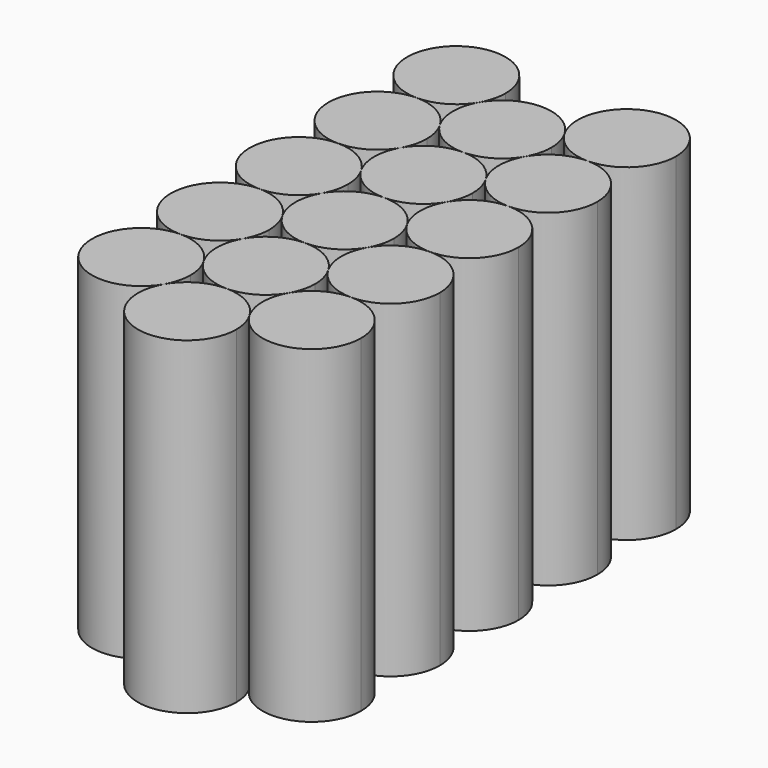
from build123d import *

# Parameters (mm, degrees)
F1_DEPTH = 70


# Not quite as in the source:
# - a feature names something its author has since deleted; it is built from what else it names


with BuildPart() as f1:
    # F0 (on Top) → F1 (new body)
    with BuildSketch(Plane.XY):
        with BuildLine():
            ThreePointArc((-9.0932666667, 5.2500001264), (-2.7176000441, -10.1422211571), (10.5, 0))
            ThreePointArc((10.5, 0), (10.1422211824, 2.71759995), (9.0932667642, 5.2499999577))
            ThreePointArc((9.0932667642, 5.2499999577), (5.2500000295, 9.0932667227), (1.93e-08, 10.5))
            ThreePointArc((1.93e-08, 10.5), (-5.2499999284, 9.0932667811), (-9.0932666667, 5.2500001264))
        make_face()
    extrude(amount=F1_DEPTH)


with BuildPart() as f1b:
    # F0 (on Top) → F1, piece 2 (new body)
    with BuildSketch(Plane.XY):
        with BuildLine():
            ThreePointArc((9.0932667504, 15.7500000185), (7.6865334795, 10.4999999862), (9.0932667642, 5.2499999577))
            ThreePointArc((9.0932667642, 5.2499999577), (20.9041334767, 0.3577788303), (28.6865334795, 10.5))
            ThreePointArc((28.6865334795, 10.5), (25.6111546956, 17.9246211888), (18.1865335182, 21))
            ThreePointArc((18.1865335182, 21), (12.9365335055, 19.5932667547), (9.0932667504, 15.7500000185))
        make_face()
    extrude(amount=F1_DEPTH)


with BuildPart() as f1c:
    # F0 (on Top) → F1, piece 3 (new body)
    with BuildSketch(Plane.XY):
        with BuildLine():
            ThreePointArc((-18.1865334408, 21), (-27.2798001924, 5.2499999535), (-9.0932666667, 5.2500001264))
            ThreePointArc((-9.0932666667, 5.2500001264), (-8.0443122845, 7.7824000969), (-7.6865334795, 10.5))
            ThreePointArc((-7.6865334795, 10.5), (-8.0443122981, 13.2175999536), (-9.0932667191, 15.7499999643))
            ThreePointArc((-9.0932667191, 15.7499999643), (-12.9365334449, 19.5932667197), (-18.1865334408, 21))
        make_face()
    extrude(amount=F1_DEPTH)


with BuildPart() as f1d:
    # F0 (on Top) → F1, piece 4 (new body)
    with BuildSketch(Plane.XY):
        with BuildLine():
            ThreePointArc((-9.0932667191, 15.7499999643), (-5.2499999738, 11.9067332451), (1.93e-08, 10.5))
            ThreePointArc((1.93e-08, 10.5), (5.2500000176, 11.9067332704), (9.0932667504, 15.7500000185))
            ThreePointArc((9.0932667504, 15.7500000185), (10.1422211788, 18.2824000367), (10.5, 21))
            ThreePointArc((10.5, 21), (10.1422211707, 23.7175999935), (9.0932667191, 26.2500000357))
            ThreePointArc((9.0932667191, 26.2500000357), (5.2499999989, 30.0932667404), (3.87e-08, 31.5))
            ThreePointArc((3.87e-08, 31.5), (-5.2500000363, 30.0932667188), (-9.093266801, 26.2499998939))
            ThreePointArc((-9.093266801, 26.2499998939), (-10.5, 20.9999999181), (-9.0932667191, 15.7499999643))
        make_face()
    extrude(amount=F1_DEPTH)


with BuildPart() as f1e:
    # F0 (on Top) → F1, piece 5 (new body)
    with BuildSketch(Plane.XY):
        with BuildLine():
            ThreePointArc((-18.1865333975, 42), (-28.6865334795, 31.5000000216), (-18.1865334408, 21))
            ThreePointArc((-18.1865334408, 21), (-12.9365335158, 22.4067332393), (-9.093266801, 26.2499998939))
            ThreePointArc((-9.093266801, 26.2499998939), (-8.0443123193, 28.7823999672), (-7.6865334795, 31.5))
            ThreePointArc((-7.6865334795, 31.5), (-8.0443123193, 34.2176000328), (-9.093266801, 36.7500001061))
            ThreePointArc((-9.093266801, 36.7500001061), (-12.9365334971, 40.5932667499), (-18.1865333975, 42))
        make_face()
    extrude(amount=F1_DEPTH)


with BuildPart() as f1f:
    # F0 (on Top) → F1, piece 6 (new body)
    with BuildSketch(Plane.XY):
        with BuildLine():
            ThreePointArc((9.0932667191, 26.2500000357), (12.9365334784, 22.4067332609), (18.1865335182, 21))
            ThreePointArc((18.1865335182, 21), (25.6111546956, 24.0753788112), (28.6865334795, 31.5))
            ThreePointArc((28.6865334795, 31.5), (25.6111547109, 38.9246211735), (18.1865335614, 42))
            ThreePointArc((18.1865335614, 42), (12.9365334971, 40.5932667499), (9.0932667191, 36.7499999643))
            ThreePointArc((9.0932667191, 36.7499999643), (7.6865334795, 31.5), (9.0932667191, 26.2500000357))
        make_face()
    extrude(amount=F1_DEPTH)


with BuildPart() as f1g:
    # F0 (on Top) → F1, piece 7 (new body)
    with BuildSketch(Plane.XY):
        with BuildLine():
            ThreePointArc((-18.1865333975, 63), (-28.6865334795, 52.5), (-18.1865333975, 42))
            ThreePointArc((-18.1865333975, 42), (-12.9365334907, 43.4067332538), (-9.0932667937, 47.2499999066))
            ThreePointArc((-9.0932667937, 47.2499999066), (-8.0443123174, 49.7823999743), (-7.6865334795, 52.5))
            ThreePointArc((-7.6865334795, 52.5), (-8.0443123193, 55.2176000328), (-9.093266801, 57.7500001061))
            ThreePointArc((-9.093266801, 57.7500001061), (-12.9365334971, 61.5932667499), (-18.1865333975, 63))
        make_face()
    extrude(amount=F1_DEPTH)


with BuildPart() as f1h:
    # F0 (on Top) → F1, piece 8 (new body)
    with BuildSketch(Plane.XY):
        with BuildLine():
            ThreePointArc((-9.0932667937, 47.2499999066), (-10.5, 42.0000000074), (-9.093266801, 36.7500001061))
            ThreePointArc((-9.093266801, 36.7500001061), (-5.2500000363, 32.9067332812), (3.87e-08, 31.5))
            ThreePointArc((3.87e-08, 31.5), (5.2499999989, 32.9067332596), (9.0932667191, 36.7499999643))
            ThreePointArc((9.0932667191, 36.7499999643), (10.1422211707, 39.2824000065), (10.5, 42))
            ThreePointArc((10.5, 42), (10.1422211838, 44.7175999446), (9.0932667697, 47.2499999481))
            ThreePointArc((9.0932667697, 47.2499999481), (5.2500000697, 51.0932666995), (1.009e-07, 52.5))
            ThreePointArc((1.009e-07, 52.5), (-5.250000003, 51.093266738), (-9.0932667937, 47.2499999066))
        make_face()
    extrude(amount=F1_DEPTH)


with BuildPart() as f1i:
    # F0 (on Top) → F1, piece 9 (new body)
    with BuildSketch(Plane.XY):
        with BuildLine():
            ThreePointArc((-18.1865333708, 84), (-28.6865334795, 73.5000000134), (-18.1865333975, 63))
            ThreePointArc((-18.1865333975, 63), (-12.9365334261, 64.4067332911), (-9.0932667191, 68.2500000357))
            ThreePointArc((-9.0932667191, 68.2500000357), (-8.0443122981, 70.7824000464), (-7.6865334795, 73.5))
            ThreePointArc((-7.6865334795, 73.5), (-8.0443122842, 76.2175999018), (-9.0932666654, 78.7499998713))
            ThreePointArc((-9.0932666654, 78.7499998713), (-12.936533368, 82.5932666754), (-18.1865333708, 84))
        make_face()
    extrude(amount=F1_DEPTH)


with BuildPart() as f1j:
    # F0 (on Top) → F1, piece 10 (new body)
    with BuildSketch(Plane.XY):
        with BuildLine():
            ThreePointArc((9.0932667697, 47.2499999481), (12.9365335409, 43.4067332248), (18.1865335614, 42))
            ThreePointArc((18.1865335614, 42), (25.6111547109, 45.0753788265), (28.6865334795, 52.5))
            ThreePointArc((28.6865334795, 52.5), (25.6111547109, 59.9246211735), (18.1865335614, 63))
            ThreePointArc((18.1865335614, 63), (12.9365334971, 61.5932667499), (9.0932667191, 57.7499999643))
            ThreePointArc((9.0932667191, 57.7499999643), (7.6865334795, 52.4999999494), (9.0932667697, 47.2499999481))
        make_face()
    extrude(amount=F1_DEPTH)


with BuildPart() as f1k:
    # F0 (on Top) → F1, piece 11 (new body)
    with BuildSketch(Plane.XY):
        with BuildLine():
            ThreePointArc((-9.0932667191, 68.2500000357), (-10.5, 63.0000000819), (-9.093266801, 57.7500001061))
            ThreePointArc((-9.093266801, 57.7500001061), (-5.2500000094, 53.9067332657), (1.009e-07, 52.5))
            ThreePointArc((1.009e-07, 52.5), (5.2500000258, 53.9067332752), (9.0932667191, 57.7499999643))
            ThreePointArc((9.0932667191, 57.7499999643), (10.1422211707, 60.2824000065), (10.5, 63))
            ThreePointArc((10.5, 63), (10.1422211953, 65.7175999018), (9.093266814, 68.2499998713))
            ThreePointArc((9.093266814, 68.2499998713), (5.249999985, 72.0932667484), (-1.832e-07, 73.5))
            ThreePointArc((-1.832e-07, 73.5), (-5.2500000615, 72.0932667042), (-9.0932667191, 68.2500000357))
        make_face()
    extrude(amount=F1_DEPTH)


with BuildPart() as f1l:
    # F0 (on Top) → F1, piece 12 (new body)
    with BuildSketch(Plane.XY):
        with BuildLine():
            ThreePointArc((-7.6865334795, 94.5), (-25.6111547204, 101.924621164), (-18.1865333708, 84))
            ThreePointArc((-18.1865333708, 84), (-12.9365334855, 85.4067332568), (-9.093266801, 89.2499998939))
            ThreePointArc((-9.093266801, 89.2499998939), (-8.0443123193, 91.7823999672), (-7.6865334795, 94.5))
        make_face()
    extrude(amount=F1_DEPTH)


with BuildPart() as f1m:
    # F0 (on Top) → F1, piece 13 (new body)
    with BuildSketch(Plane.XY):
        with BuildLine():
            ThreePointArc((-9.093266801, 89.2499998939), (-10.5, 83.9999998644), (-9.0932666654, 78.7499998713))
            ThreePointArc((-9.0932666654, 78.7499998713), (-5.250000015, 74.9067332689), (-1.832e-07, 73.5))
            ThreePointArc((-1.832e-07, 73.5), (5.2499999385, 74.9067332248), (9.0932667604, 78.7500000357))
            ThreePointArc((9.0932667604, 78.7500000357), (10.1422211814, 81.2824000464), (10.5, 84))
            ThreePointArc((10.5, 84), (10.1422211739, 86.7175999816), (9.0932667315, 89.2500000143))
            ThreePointArc((9.0932667315, 89.2500000143), (-6.95e-08, 94.5), (-9.093266801, 89.2499998939))
        make_face()
    extrude(amount=F1_DEPTH)


with BuildPart() as f1n:
    # F0 (on Top) → F1, piece 14 (new body)
    with BuildSketch(Plane.XY):
        with BuildLine():
            ThreePointArc((9.093266814, 68.2499998713), (12.9365335793, 64.4067332026), (18.1865335614, 63))
            ThreePointArc((18.1865335614, 63), (25.6111547109, 66.0753788265), (28.6865334795, 73.5))
            ThreePointArc((28.6865334795, 73.5), (25.6111547119, 80.9246211725), (18.1865335643, 84))
            ThreePointArc((18.1865335643, 84), (12.9365335341, 82.5932667713), (9.0932667604, 78.7500000357))
            ThreePointArc((9.0932667604, 78.7500000357), (7.6865334795, 73.4999999463), (9.093266814, 68.2499998713))
        make_face()
    extrude(amount=F1_DEPTH)


with BuildPart() as f1o:
    # F0 (on Top) → F1, piece 15 (new body)
    with BuildSketch(Plane.XY):
        with BuildLine():
            ThreePointArc((28.6865334795, 94.5), (15.4689335139, 104.6422211782), (9.0932667315, 89.2500000143))
            ThreePointArc((9.0932667315, 89.2500000143), (12.9365335091, 85.4067332432), (18.1865335643, 84))
            ThreePointArc((18.1865335643, 84), (25.6111547119, 87.0753788275), (28.6865334795, 94.5))
        make_face()
    extrude(amount=F1_DEPTH)


solid = Compound([f1.part, f1b.part, f1c.part, f1d.part, f1e.part, f1f.part, f1g.part, f1h.part, f1i.part, f1j.part, f1k.part, f1l.part, f1m.part, f1n.part, f1o.part])
